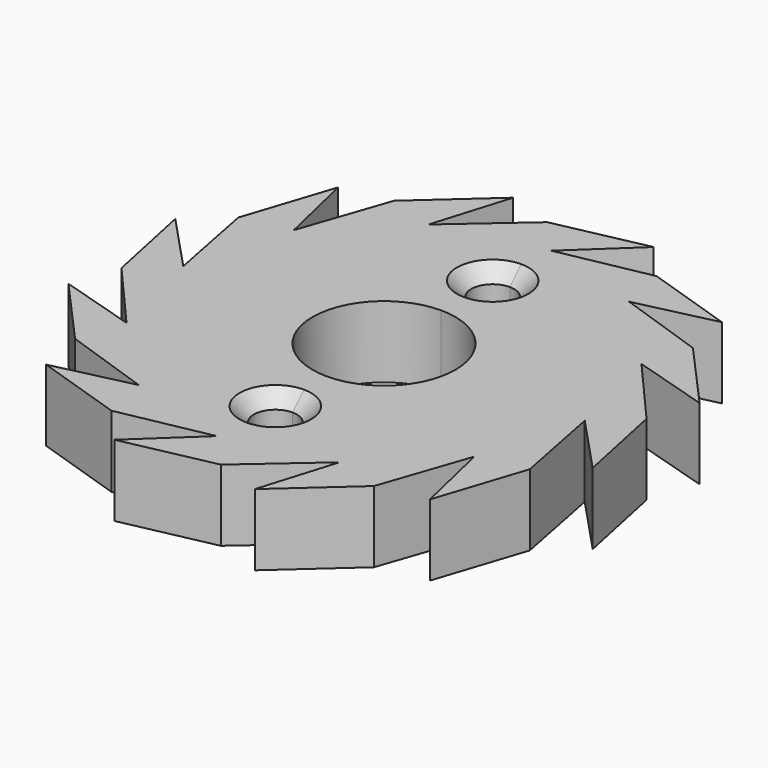
from build123d import *

# Parameters (mm, degrees)
F1_DEPTH = 6.35
F2_SIZE  = 1.27


# Not quite as in the source:
# - a feature names something its author has since deleted; it is built from what else it names


with BuildPart() as f1:
    # F0 (on Top) → F1 (new body)
    with BuildSketch(Plane.XY):
        with BuildLine():
            ThreePointArc((16.2360474276, -7.2470106892), (17.3897286244, -3.7048263615), (17.78, 0))
            ThreePointArc((17.78, 0), (17.7560676116, 0.9222054927), (17.6843348739, 1.8419283555))
            ThreePointArc((17.6843348739, 1.8419283555), (16.9123599344, 5.4863905666), (15.3979316793, 8.89))
            ThreePointArc((15.3979316793, 8.89), (14.9161028766, 9.67668719), (14.3941190721, 10.4373241848))
            ThreePointArc((14.3941190721, 10.4373241848), (11.9033380579, 13.2075335729), (8.89, 15.3979316793))
            ThreePointArc((8.89, 15.3979316793), (8.0793804216, 15.8383083694), (7.2470106892, 16.2360474276))
            ThreePointArc((7.2470106892, 16.2360474276), (3.7048263615, 17.3897286244), (0, 17.78))
            Line((0, 17.78), (0, 13.97))
            ThreePointArc((0, 13.97), (1.3470384182, 13.4120384182), (1.905, 12.065))
            ThreePointArc((1.905, 12.065), (1.3470384182, 10.7179615818), (0, 10.16))
            Line((0, 10.16), (0, 6.35))
            ThreePointArc((0, 6.35), (4.4901280605, 4.4901280605), (6.35, 0))
            ThreePointArc((6.35, 0), (4.4901280605, -4.4901280605), (0, -6.35))
            Line((0, -6.35), (0, -10.16))
            ThreePointArc((0, -10.16), (1.3470384182, -10.7179615818), (1.905, -12.065))
            ThreePointArc((1.905, -12.065), (1.3470384182, -13.4120384182), (0, -13.97))
            Line((0, -13.97), (0, -17.78))
            ThreePointArc((0, -17.78), (0.9222054927, -17.7560676116), (1.8419283555, -17.6843348739))
            ThreePointArc((1.8419283555, -17.6843348739), (5.4863905666, -16.9123599344), (8.89, -15.3979316793))
            ThreePointArc((8.89, -15.3979316793), (9.67668719, -14.9161028766), (10.4373241848, -14.3941190721))
            ThreePointArc((10.4373241848, -14.3941190721), (13.2075335729, -11.9033380579), (15.3979316793, -8.89))
            ThreePointArc((15.3979316793, -8.89), (15.8383083694, -8.0793804216), (16.2360474276, -7.2470106892))
        make_face()
        with BuildLine():
            Line((18.1161912512, -0.3593002622), (17.78, 0))
            ThreePointArc((17.78, 0), (17.3897286244, -3.7048263615), (16.2360474276, -7.2470106892))
            Line((16.2360474276, -7.2470106892), (15.5094317122, -9.3692587802))
            Line((15.5094317122, -9.3692587802), (17.1246183088, -16.3117890891))
            Line((17.1246183088, -16.3117890891), (19.7021180322, -8.4429771511))
            Line((19.7021180322, -8.4429771511), (18.1161912512, -0.3593002622))
        make_face()
        with BuildLine():
            ThreePointArc((17.6843348739, 1.8419283555), (17.7560676116, 0.9222054927), (17.78, 0))
            Line((17.78, 0), (18.1161912512, -0.3593002622))
            Line((18.1161912512, -0.3593002622), (17.6843348739, 1.8419283555))
        make_face()
        with BuildLine():
            ThreePointArc((15.3979316793, 8.89), (16.9123599344, 5.4863905666), (17.6843348739, 1.8419283555))
            Line((17.6843348739, 1.8419283555), (18.1161912512, -0.3593002622))
            Line((18.1161912512, -0.3593002622), (22.9862490301, -5.564114578))
            Line((22.9862490301, -5.564114578), (21.2840232998, 2.5392263196))
            Line((21.2840232998, 2.5392263196), (15.8687319744, 8.7469324709))
            Line((15.8687319744, 8.7469324709), (15.3979316793, 8.89))
        make_face()
        with BuildLine():
            Line((15.5094317122, -9.3692587802), (16.2360474276, -7.2470106892))
            ThreePointArc((16.2360474276, -7.2470106892), (15.8383083694, -8.0793804216), (15.3979316793, -8.89))
            Line((15.3979316793, -8.89), (15.5094317122, -9.3692587802))
        make_face()
        with BuildLine():
            ThreePointArc((14.3941190721, 10.4373241848), (14.9161028766, 9.67668719), (15.3979316793, 8.89))
            Line((15.3979316793, 8.89), (15.8687319744, 8.7469324709))
            Line((15.8687319744, 8.7469324709), (14.3941190721, 10.4373241848))
        make_face()
        with BuildLine():
            Line((15.5094317122, -9.3692587802), (15.3979316793, -8.89))
            ThreePointArc((15.3979316793, -8.89), (13.2075335729, -11.9033380579), (10.4373241848, -14.3941190721))
            Line((10.4373241848, -14.3941190721), (8.7469324709, -15.8687319744))
            Line((8.7469324709, -15.8687319744), (6.674459941, -22.6887328868))
            Line((6.674459941, -22.6887328868), (12.8410461487, -17.1628917126))
            Line((12.8410461487, -17.1628917126), (15.5094317122, -9.3692587802))
        make_face()
        with BuildLine():
            ThreePointArc((8.89, 15.3979316793), (11.9033380579, 13.2075335729), (14.3941190721, 10.4373241848))
            Line((14.3941190721, 10.4373241848), (15.8687319744, 8.7469324709))
            Line((15.8687319744, 8.7469324709), (22.6887328868, 6.674459941))
            Line((22.6887328868, 6.674459941), (17.1628917126, 12.8410461487))
            Line((17.1628917126, 12.8410461487), (9.3692587802, 15.5094317122))
            Line((9.3692587802, 15.5094317122), (8.89, 15.3979316793))
        make_face()
        with BuildLine():
            Line((8.7469324709, -15.8687319744), (10.4373241848, -14.3941190721))
            ThreePointArc((10.4373241848, -14.3941190721), (9.67668719, -14.9161028766), (8.89, -15.3979316793))
            Line((8.89, -15.3979316793), (8.7469324709, -15.8687319744))
        make_face()
        with BuildLine():
            ThreePointArc((7.2470106892, 16.2360474276), (8.0793804216, 15.8383083694), (8.89, 15.3979316793))
            Line((8.89, 15.3979316793), (9.3692587802, 15.5094317122))
            Line((9.3692587802, 15.5094317122), (7.2470106892, 16.2360474276))
        make_face()
        with BuildLine():
            Line((8.7469324709, -15.8687319744), (8.89, -15.3979316793))
            ThreePointArc((8.89, -15.3979316793), (5.4863905666, -16.9123599344), (1.8419283555, -17.6843348739))
            Line((1.8419283555, -17.6843348739), (-0.3593002622, -18.1161912512))
            Line((-0.3593002622, -18.1161912512), (-5.564114578, -22.9862490301))
            Line((-5.564114578, -22.9862490301), (2.5392263196, -21.2840232998))
            Line((2.5392263196, -21.2840232998), (8.7469324709, -15.8687319744))
        make_face()
        with BuildLine():
            ThreePointArc((0, 17.78), (3.7048263615, 17.3897286244), (7.2470106892, 16.2360474276))
            Line((7.2470106892, 16.2360474276), (9.3692587802, 15.5094317122))
            Line((9.3692587802, 15.5094317122), (16.3117890891, 17.1246183088))
            Line((16.3117890891, 17.1246183088), (8.4429771511, 19.7021180322))
            Line((8.4429771511, 19.7021180322), (0.3593002622, 18.1161912512))
            Line((0.3593002622, 18.1161912512), (0, 17.78))
        make_face()
        with BuildLine():
            Line((-0.3593002622, -18.1161912512), (1.8419283555, -17.6843348739))
            ThreePointArc((1.8419283555, -17.6843348739), (0.9222054927, -17.7560676116), (0, -17.78))
            Line((0, -17.78), (-0.3593002622, -18.1161912512))
        make_face()
        with BuildLine():
            Line((0, 13.97), (0, 17.78))
            ThreePointArc((0, 17.78), (-0.9222054927, 17.7560676116), (-1.8419283555, 17.6843348739))
            ThreePointArc((-1.8419283555, 17.6843348739), (-5.4863905666, 16.9123599344), (-8.89, 15.3979316793))
            ThreePointArc((-8.89, 15.3979316793), (-9.67668719, 14.9161028766), (-10.4373241848, 14.3941190721))
            ThreePointArc((-10.4373241848, 14.3941190721), (-13.2075335729, 11.9033380579), (-15.3979316793, 8.89))
            ThreePointArc((-15.3979316793, 8.89), (-15.8383083694, 8.0793804216), (-16.2360474276, 7.2470106892))
            ThreePointArc((-16.2360474276, 7.2470106892), (-17.3897286244, 3.7048263615), (-17.78, 0))
            ThreePointArc((-17.78, 0), (-17.7560676116, -0.9222054927), (-17.6843348739, -1.8419283555))
            ThreePointArc((-17.6843348739, -1.8419283555), (-16.9123599344, -5.4863905666), (-15.3979316793, -8.89))
            ThreePointArc((-15.3979316793, -8.89), (-14.9161028766, -9.67668719), (-14.3941190721, -10.4373241848))
            ThreePointArc((-14.3941190721, -10.4373241848), (-11.9033380579, -13.2075335729), (-8.89, -15.3979316793))
            ThreePointArc((-8.89, -15.3979316793), (-8.0793804216, -15.8383083694), (-7.2470106892, -16.2360474276))
            ThreePointArc((-7.2470106892, -16.2360474276), (-3.7048263615, -17.3897286244), (0, -17.78))
            Line((0, -17.78), (0, -13.97))
            ThreePointArc((0, -13.97), (-1.905, -12.065), (0, -10.16))
            Line((0, -10.16), (0, -6.35))
            ThreePointArc((0, -6.35), (-6.35, 0), (0, 6.35))
            Line((0, 6.35), (0, 10.16))
            ThreePointArc((0, 10.16), (-1.905, 12.065), (0, 13.97))
        make_face()
        with BuildLine():
            ThreePointArc((-1.8419283555, 17.6843348739), (-0.9222054927, 17.7560676116), (0, 17.78))
            Line((0, 17.78), (0.3593002622, 18.1161912512))
            Line((0.3593002622, 18.1161912512), (-1.8419283555, 17.6843348739))
        make_face()
        with BuildLine():
            Line((-0.3593002622, -18.1161912512), (0, -17.78))
            ThreePointArc((0, -17.78), (-3.7048263615, -17.3897286244), (-7.2470106892, -16.2360474276))
            Line((-7.2470106892, -16.2360474276), (-9.3692587802, -15.5094317122))
            Line((-9.3692587802, -15.5094317122), (-16.3117890891, -17.1246183088))
            Line((-16.3117890891, -17.1246183088), (-8.4429771511, -19.7021180322))
            Line((-8.4429771511, -19.7021180322), (-0.3593002622, -18.1161912512))
        make_face()
        with BuildLine():
            ThreePointArc((-8.89, 15.3979316793), (-5.4863905666, 16.9123599344), (-1.8419283555, 17.6843348739))
            Line((-1.8419283555, 17.6843348739), (0.3593002622, 18.1161912512))
            Line((0.3593002622, 18.1161912512), (5.564114578, 22.9862490301))
            Line((5.564114578, 22.9862490301), (-2.5392263196, 21.2840232998))
            Line((-2.5392263196, 21.2840232998), (-8.7469324709, 15.8687319744))
            Line((-8.7469324709, 15.8687319744), (-8.89, 15.3979316793))
        make_face()
        with BuildLine():
            Line((-9.3692587802, -15.5094317122), (-7.2470106892, -16.2360474276))
            ThreePointArc((-7.2470106892, -16.2360474276), (-8.0793804216, -15.8383083694), (-8.89, -15.3979316793))
            Line((-8.89, -15.3979316793), (-9.3692587802, -15.5094317122))
        make_face()
        with BuildLine():
            ThreePointArc((-10.4373241848, 14.3941190721), (-9.67668719, 14.9161028766), (-8.89, 15.3979316793))
            Line((-8.89, 15.3979316793), (-8.7469324709, 15.8687319744))
            Line((-8.7469324709, 15.8687319744), (-10.4373241848, 14.3941190721))
        make_face()
        with BuildLine():
            Line((-9.3692587802, -15.5094317122), (-8.89, -15.3979316793))
            ThreePointArc((-8.89, -15.3979316793), (-11.9033380579, -13.2075335729), (-14.3941190721, -10.4373241848))
            Line((-14.3941190721, -10.4373241848), (-15.8687319744, -8.7469324709))
            Line((-15.8687319744, -8.7469324709), (-22.6887328868, -6.674459941))
            Line((-22.6887328868, -6.674459941), (-17.1628917126, -12.8410461487))
            Line((-17.1628917126, -12.8410461487), (-9.3692587802, -15.5094317122))
        make_face()
        with BuildLine():
            ThreePointArc((-15.3979316793, 8.89), (-13.2075335729, 11.9033380579), (-10.4373241848, 14.3941190721))
            Line((-10.4373241848, 14.3941190721), (-8.7469324709, 15.8687319744))
            Line((-8.7469324709, 15.8687319744), (-6.674459941, 22.6887328868))
            Line((-6.674459941, 22.6887328868), (-12.8410461487, 17.1628917126))
            Line((-12.8410461487, 17.1628917126), (-15.5094317122, 9.3692587802))
            Line((-15.5094317122, 9.3692587802), (-15.3979316793, 8.89))
        make_face()
        with BuildLine():
            Line((-15.8687319744, -8.7469324709), (-14.3941190721, -10.4373241848))
            ThreePointArc((-14.3941190721, -10.4373241848), (-14.9161028766, -9.67668719), (-15.3979316793, -8.89))
            Line((-15.3979316793, -8.89), (-15.8687319744, -8.7469324709))
        make_face()
        with BuildLine():
            ThreePointArc((-16.2360474276, 7.2470106892), (-15.8383083694, 8.0793804216), (-15.3979316793, 8.89))
            Line((-15.3979316793, 8.89), (-15.5094317122, 9.3692587802))
            Line((-15.5094317122, 9.3692587802), (-16.2360474276, 7.2470106892))
        make_face()
        with BuildLine():
            Line((-15.8687319744, -8.7469324709), (-15.3979316793, -8.89))
            ThreePointArc((-15.3979316793, -8.89), (-16.9123599344, -5.4863905666), (-17.6843348739, -1.8419283555))
            Line((-17.6843348739, -1.8419283555), (-18.1161912512, 0.3593002622))
            Line((-18.1161912512, 0.3593002622), (-22.9862490301, 5.564114578))
            Line((-22.9862490301, 5.564114578), (-21.2840232998, -2.5392263196))
            Line((-21.2840232998, -2.5392263196), (-15.8687319744, -8.7469324709))
        make_face()
        with BuildLine():
            ThreePointArc((-17.78, 0), (-17.3897286244, 3.7048263615), (-16.2360474276, 7.2470106892))
            Line((-16.2360474276, 7.2470106892), (-15.5094317122, 9.3692587802))
            Line((-15.5094317122, 9.3692587802), (-17.1246183088, 16.3117890891))
            Line((-17.1246183088, 16.3117890891), (-19.7021180322, 8.4429771511))
            Line((-19.7021180322, 8.4429771511), (-18.1161912512, 0.3593002622))
            Line((-18.1161912512, 0.3593002622), (-17.78, 0))
        make_face()
        with BuildLine():
            Line((-18.1161912512, 0.3593002622), (-17.6843348739, -1.8419283555))
            ThreePointArc((-17.6843348739, -1.8419283555), (-17.7560676116, -0.9222054927), (-17.78, 0))
            Line((-17.78, 0), (-18.1161912512, 0.3593002622))
        make_face()
    extrude(amount=F1_DEPTH)

    # F2
    f2_edges = [f1.edges().sort_by_distance(p)[0] for p in [
        (-1.905, 12.065, 6.35),
        (-1.905, -12.065, 6.35),
    ]]
    chamfer(f2_edges, length=F2_SIZE)


solid = f1.part
